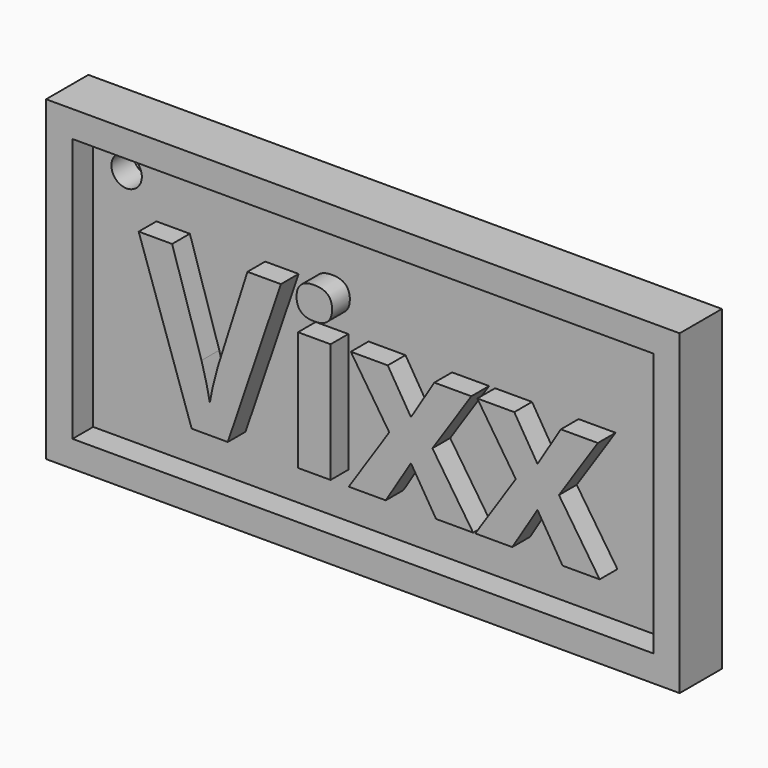
from build123d import *

# Parameters (mm, degrees)
F0_TEXT_SIZE = 26.3212435233
F1_DEPTH     = 5.9055
F0_W         = 76.2
F0_H         = 38.1
F0_W_2       = 69.85
F0_H_2       = 31.75
F2_DEPTH     = 6.35
F0_W_3       = 3.9193976684
F0_H_3       = 14.369753886
F0_R         = 1.8297536171
F3_DEPTH     = 3.2385


# Not quite as in the source:
# - Text() gives the source's letters only with a copy of the font that has no kerning and outlines rounded to 1/6400 em; it was checked with that copy


with BuildPart() as f1:
    # F0 (on Front) → F1 (new body)
    with BuildSketch(Plane.XZ):
        with Locations((-28.575, -2.7293343303)):
            Text('Vixx', F0_TEXT_SIZE, font='Open Sans', font_style=FontStyle.BOLD, text_align=(TextAlign.LEFT, TextAlign.BOTTOM))
    extrude(amount=F1_DEPTH)


with BuildPart() as f2:
    # F0 (on Front) → F2 (new body)
    with BuildSketch(Plane.XZ):
        with Locations((-1.2546796352, 7.7012310267)):
            Rectangle(F0_W, F0_H)
        with Locations((-1.2546796352, 7.7012310267)):
            Rectangle(F0_W_2, F0_H_2, mode=Mode.SUBTRACT)
    extrude(amount=F2_DEPTH)


with BuildPart() as f3:
    # F0 (on Front) → F3 (new body)
    with BuildSketch(Plane.XZ):
        with Locations((-1.2546796352, 7.7012310267)):
            Rectangle(F0_W_2, F0_H_2)
        with BuildLine():
            Line((-19.05, 4.8791501257), (-15.4925194301, 16.0615659288))
            Line((-15.4925194301, 16.0615659288), (-11.4703044041, 16.0615659288))
            Line((-11.4703044041, 16.0615659288), (-17.8573186528, -2.7293343303))
            Line((-17.8573186528, -2.7293343303), (-22.2003238342, -2.7293343303))
            Line((-22.2003238342, -2.7293343303), (-28.575, 16.0615659288))
            Line((-28.575, 16.0615659288), (-24.5527849741, 16.0615659288))
            Line((-24.5527849741, 16.0615659288), (-21.0158678756, 4.8791501257))
            add(Edge.make_bspline(
                [(-21.0158678756, 4.8791501257), (-20.7238665803, 3.8879907993), (-20.4071891192, 2.5719286231)],
                knots=[0, 0, 0, 1, 1, 1], degree=2))
            add(Edge.make_bspline(
                [(-20.4071891192, 2.5719286231), (-20.090511658, 1.2558664469), (-20.0164831606, 0.7417796594)],
                knots=[0, 0, 0, 1, 1, 1], degree=2))
            add(Edge.make_bspline(
                [(-20.0164831606, 0.7417796594), (-19.8725388601, 1.9221229236), (-19.05, 4.8791501257)],
                knots=[0, 0, 0, 1, 1, 1], degree=2))
        make_face(mode=Mode.SUBTRACT)
        with Locations((-7.4542584197, 4.4555426127)):
            Rectangle(F0_W_3, F0_H_3, mode=Mode.SUBTRACT)
        Polygon((-3.3107189119, -2.7293343303), (1.5628238342, 4.6077123019), (-3.0639572539, 11.6404195557), (1.381865285, 11.6404195557), (4.1702720207, 7.0629907993), (6.9833549223, 11.6404195557), (11.4332901554, 11.6404195557), (6.7530440415, 4.6077123019), (11.6512629534, -2.7293343303), (7.1889896373, -2.7293343303), (4.1702720207, 2.1935607475), (1.1392163212, -2.7293343303), align=None, mode=Mode.SUBTRACT)
        Polygon((11.90625, -2.7293343303), (16.7797927461, 4.6077123019), (12.153011658, 11.6404195557), (16.5988341969, 11.6404195557), (19.3872409326, 7.0629907993), (22.2003238342, 11.6404195557), (26.6502590674, 11.6404195557), (21.9700129534, 4.6077123019), (26.8682318653, -2.7293343303), (22.4059585492, -2.7293343303), (19.3872409326, 2.1935607475), (16.3561852332, -2.7293343303), align=None, mode=Mode.SUBTRACT)
        with BuildLine():
            add(Edge.make_bspline(
                [(-7.4480893782, 13.4253288822), (-9.5825777202, 13.4253288822), (-9.5825777202, 15.3541825091)],
                knots=[0, 0, 0, 1, 1, 1], degree=2))
            add(Edge.make_bspline(
                [(-9.5825777202, 15.3541825091), (-9.5825777202, 17.2706980532), (-7.4480893782, 17.2706980532)],
                knots=[0, 0, 0, 1, 1, 1], degree=2))
            add(Edge.make_bspline(
                [(-7.4480893782, 17.2706980532), (-5.3136010363, 17.2706980532), (-5.3136010363, 15.3541825091)],
                knots=[0, 0, 0, 1, 1, 1], degree=2))
            add(Edge.make_bspline(
                [(-5.3136010363, 15.3541825091), (-5.3136010363, 14.4411643744), (-5.8461949482, 13.9332466283)],
                knots=[0, 0, 0, 1, 1, 1], degree=2))
            add(Edge.make_bspline(
                [(-5.8461949482, 13.9332466283), (-6.3787888601, 13.4253288822), (-7.4480893782, 13.4253288822)],
                knots=[0, 0, 0, 1, 1, 1], degree=2))
        make_face(mode=Mode.SUBTRACT)
        with Locations((-32.1572758257, 20.2136002481)):
            Circle(F0_R, mode=Mode.SUBTRACT)
    extrude(amount=F3_DEPTH)


solid = Compound([f1.part, f2.part, f3.part])
